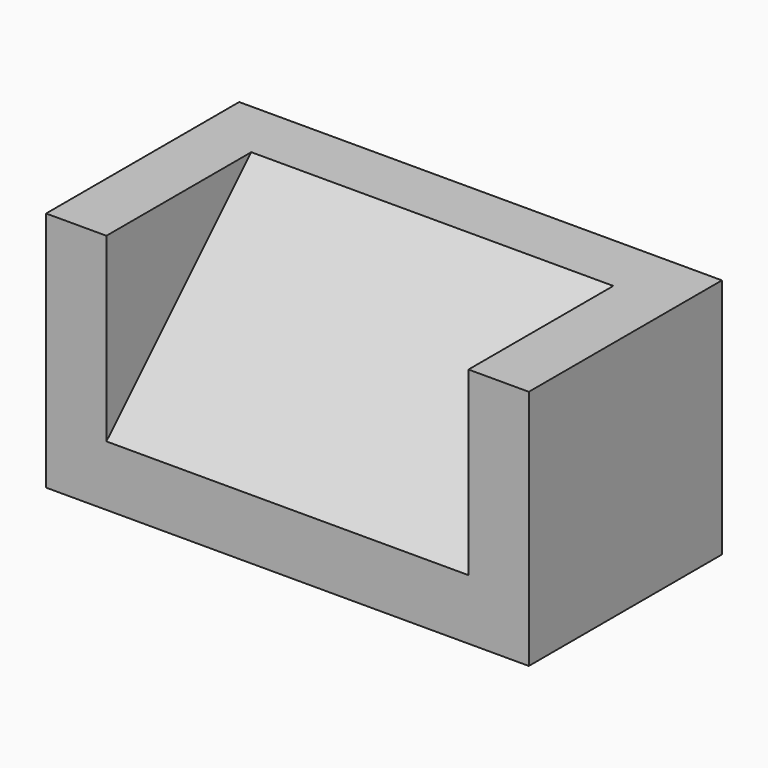
from build123d import *

# Parameters (mm, degrees)
F1_DEPTH = 101.6
F0_W     = 152.4
F0_H     = 76.2
F2_DEPTH = 25.4
F3_DEPTH = 76.2
F4_SIZE  = 76.19999


# Not quite as in the source:
# - a fillet or chamfer is up to 0.001 mm smaller than in the source, because OpenCascade refuses the exact size


with BuildPart() as f1:
    # F0 (on Front) → F1 (new body)
    with BuildSketch(Plane.XZ):
        Polygon((-152.4, 0), (0, 0), (25.4, 0), (25.4, 101.6), (0, 101.6), (0, 25.4), (-152.4, 25.4), (-152.4, 101.6), (-177.8, 101.6), (-177.8, 0), align=None)
    extrude(amount=F1_DEPTH)

    # F0 (on Front) → F2 (join)
    with BuildSketch(Plane.XZ):
        with Locations((-76.2, 63.5)):
            Rectangle(F0_W, F0_H)
    extrude(amount=F2_DEPTH)


with BuildPart() as f3:
    # F3 (new): a face of the model
    f3_faces = [f1.part.faces().sort_by_distance(p)[0] for p in [
        (-76.2, -25.4, 63.5),
    ]]
    extrude(f3_faces, amount=F3_DEPTH)

    # F4 (size 76.2 in the source; OpenCascade refuses exactly that, so slightly less here)
    f4_edges = [f3.edges().sort_by_distance(p)[0] for p in [
        (-76.2, -101.6, 101.6),
    ]]
    chamfer(f4_edges, length=F4_SIZE)


solid = Compound([f1.part, f3.part])
